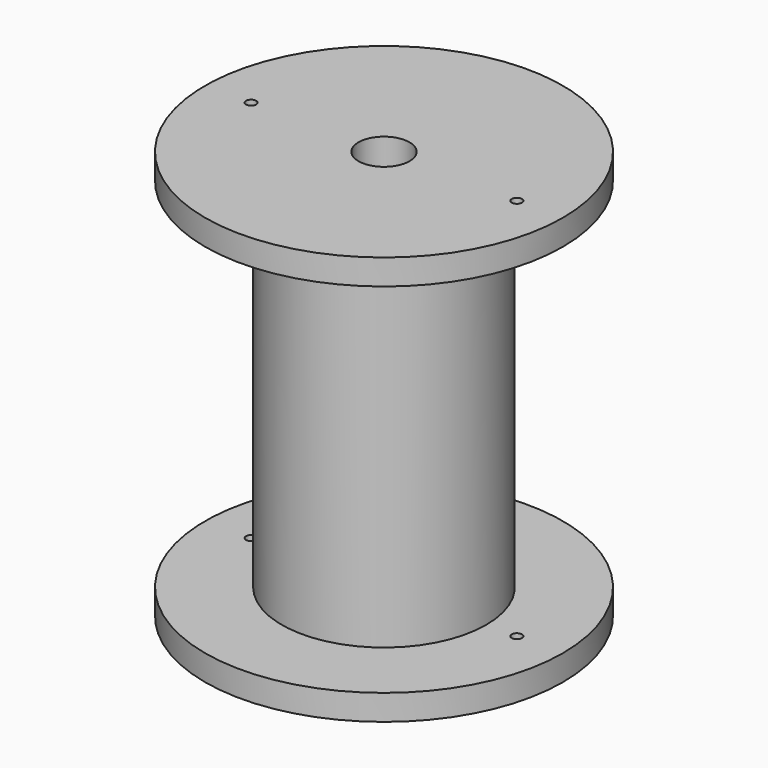
from build123d import *

# Parameters (mm, degrees)
F0_R     = 22.225
F1_DEPTH = 3.175
F2_R     = 12.7
F3_DEPTH = 44.45
F4_R     = 22.225
F5_DEPTH = 3.175
F6_R     = 0.635
F7_DEPTH = 50.8
F8_T     = -1.778


# Not quite as in the source:
# - a length typed as a fraction of an inch, garbled in the dataset ("3 / 203.2 mm" for 3/8 in), is restored


with BuildPart() as f1:
    # F0 (on Top) → F1 (new body)
    with BuildSketch(Plane.XY):
        Circle(F0_R)
    extrude(amount=F1_DEPTH)

    # F2 (on face) → F3 (join)
    with BuildSketch(Plane(origin=(0, 0, 0), x_dir=(1, 0, 0), z_dir=(0, 0, -1))):
        Circle(F2_R)
    extrude(amount=F3_DEPTH)

    # F4 (on face) → F5 (join)
    with BuildSketch(Plane(origin=(0, 0, -44.45), x_dir=(1, 0, 0), z_dir=(0, 0, -1))):
        Circle(F4_R)
    extrude(amount=F5_DEPTH)

    # F6 (on face) → F7 (cut, through all)
    with BuildSketch(Plane.XY.offset(3.175)):
        with BuildLine():
            ThreePointArc((-3.175, 0), (0, -3.175), (3.175, 0))
            ThreePointArc((3.175, 0), (0, 3.175), (-3.175, 0))
        make_face()
        with BuildLine():
            ThreePointArc((-17.145, 0), (-16.51, -0.635), (-15.875, 0))
            Line((-15.875, 0), (-17.145, 0))
        make_face()
        with BuildLine():
            Line((-17.145, 0), (-15.875, 0))
            ThreePointArc((-15.875, 0), (-16.51, 0.635), (-17.145, 0))
        make_face()
        with Locations((16.51, 0)):
            Circle(F6_R)
    extrude(amount=-F7_DEPTH, mode=Mode.SUBTRACT)

    # F8 (hollow: no face is removed)
    offset(amount=F8_T, kind=Kind.INTERSECTION, mode=Mode.SUBTRACT)


solid = f1.part
